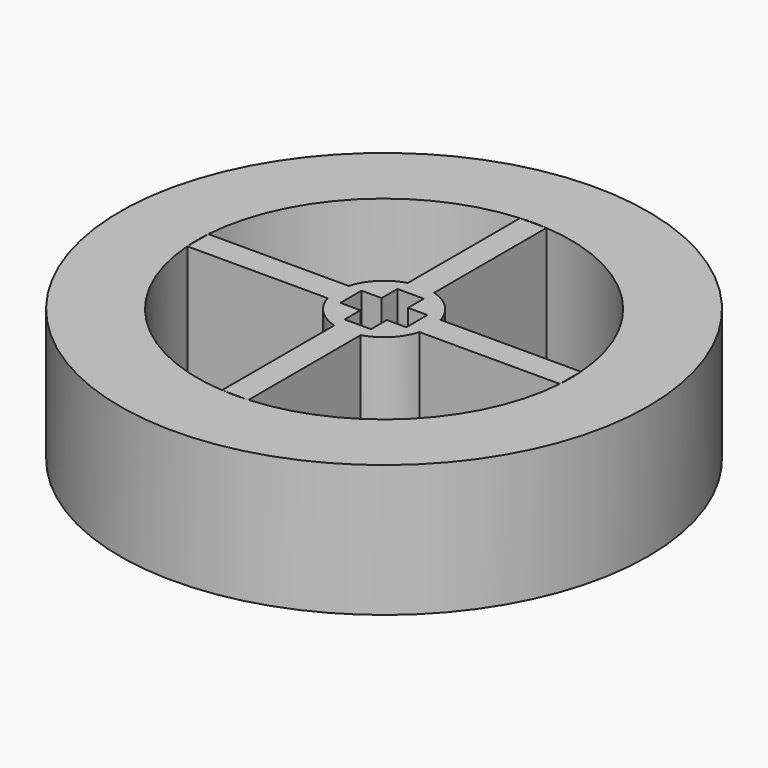
from build123d import *

# Parameters (mm, degrees)
F1_R     = 3.619217407
F2_DEPTH = 10
F0_W     = 2
F0_H     = 2
F0_W_2   = 1.4766840935
F0_H_2   = 1.5
F0_W_3   = 1.5233159065
F3_DEPTH = 10
F5_DEPTH = 10
F4_R     = 19.9994931562


# Not quite as in the source:
# - a feature names something its author has since deleted; it is built from what else it names


with BuildPart() as f2:
    # F1 (on Top) → F2 (new body)
    with BuildSketch(Plane.XY):
        Circle(F1_R)
    extrude(amount=F2_DEPTH)

    # F0 (on Top) → F3 (cut)
    with BuildSketch(Plane.XY):
        with Locations((0.0116579533, 0)):
            Rectangle(F0_W, F0_H)
        with Locations((1.75, 0)):
            Rectangle(F0_W_2, F0_H)
        with Locations((0.0116579533, -1.75)):
            Rectangle(F0_W, F0_H_2)
        with Locations((0.0116579533, 1.75)):
            Rectangle(F0_W, F0_H_2)
        with Locations((-1.75, 0)):
            Rectangle(F0_W_3, F0_H)
    extrude(amount=F3_DEPTH, mode=Mode.SUBTRACT)

    # F4 (on face) → F5 (join)
    with BuildSketch(Plane.XY.offset(10)):
        with BuildLine():
            Line((1.0116579533, 3.4749507658), (1.0116579533, 14.1129590508))
            Line((1.0116579533, 14.1129590508), (-0.9883420467, 14.1146110461))
            Line((-0.9883420467, 14.1146110461), (-0.9883420467, 3.4816540089))
            ThreePointArc((-0.9883420467, 3.4816540089), (0.0121301789, 3.6191970791), (1.0116579533, 3.4749507658))
        make_face()
        with BuildLine():
            Line((14.1137898874, -1), (14.1137898874, 1))
            Line((14.1137898874, 1), (3.4783235385, 1))
            ThreePointArc((3.4783235385, 1), (3.5838208477, 0.5049383829), (3.619217407, 0))
            ThreePointArc((3.619217407, 0), (3.5838208477, -0.5049383829), (3.4783235385, -1))
            Line((3.4783235385, -1), (14.1137898874, -1))
        make_face()
        with BuildLine():
            Line((-0.9883420467, -14.1146110461), (1.0116579533, -14.1129590508))
            Line((1.0116579533, -14.1129590508), (1.0116579533, -3.4749507658))
            ThreePointArc((1.0116579533, -3.4749507658), (0.0121301789, -3.6191970791), (-0.9883420467, -3.4816540089))
            Line((-0.9883420467, -3.4816540089), (-0.9883420467, -14.1146110461))
        make_face()
        with BuildLine():
            Line((-3.4783235385, 1), (-14.1137898874, 1))
            Line((-14.1137898874, 1), (-14.1137898874, -1))
            Line((-14.1137898874, -1), (-3.4783235385, -1))
            ThreePointArc((-3.4783235385, -1), (-3.619217407, 0), (-3.4783235385, 1))
        make_face()
    extrude(amount=-F5_DEPTH)

    # F4 (on face) → F5, piece 2 (join)
    with BuildSketch(Plane.XY.offset(10)):
        Circle(F4_R)
        with BuildLine():
            ThreePointArc((14.1137898874, 1), (14.1403236177, 0.5003128735), (14.1491718833, 0))
            ThreePointArc((14.1491718833, 0), (14.1403236177, -0.5003128735), (14.1137898874, -1))
            ThreePointArc((14.1137898874, -1), (10.0091066965, -10.0008423706), (1.0116579533, -14.1129590508))
            ThreePointArc((1.0116579533, -14.1129590508), (0.0116871787, -14.1491670566), (-0.9883420467, -14.1146110461))
            ThreePointArc((-0.9883420467, -14.1146110461), (-10.0008426126, -10.0091064548), (-14.1137898874, -1))
            ThreePointArc((-14.1137898874, -1), (-14.1491718833, 0), (-14.1137898874, 1))
            ThreePointArc((-14.1137898874, 1), (-10.0008426126, 10.0091064548), (-0.9883420467, 14.1146110461))
            ThreePointArc((-0.9883420467, 14.1146110461), (0.0116871787, 14.1491670566), (1.0116579533, 14.1129590508))
            ThreePointArc((1.0116579533, 14.1129590508), (10.0091066965, 10.0008423706), (14.1137898874, 1))
        make_face(mode=Mode.SUBTRACT)
    extrude(amount=-F5_DEPTH)


solid = f2.part
